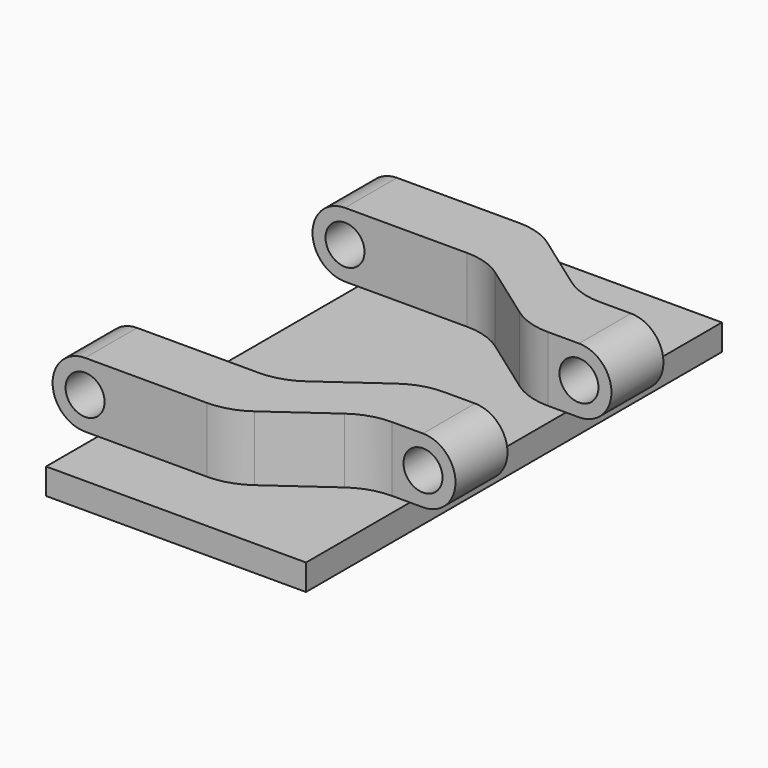
from build123d import *

# Parameters (mm, degrees)
F0_W          = 20
F0_H          = 1
F1_DEPTH      = 20
F1_DEPTH_BACK = 20
F3_DEPTH      = 40
F5_DEPTH      = 5
F7_R          = 1.5
F8_DEPTH      = 20.001
F8_DEPTH_BACK = 20.001
F9_R          = 5


# Not quite as in the source:
# - a pattern or mirror of a feature is missing from the dataset's text; its kind, count and spacing are read off the source's solid


with BuildPart() as f1:
    # F0 (on Front) → F1 (new body, two sides)
    with BuildSketch(Plane.XZ) as f1_sk:
        with Locations((0, -0.5)):
            Rectangle(F0_W, F0_H)
    extrude(amount=F1_DEPTH)
    extrude(f1_sk.sketch, amount=-F1_DEPTH_BACK)

    # F2 (on face) → F3 (join, through all)
    with BuildSketch(Plane(origin=(0, 20, 0), x_dir=(-1, 0, 0), z_dir=(0, 1, 0))):
        with BuildLine():
            Line((10, 1), (11, 1))
            ThreePointArc((11, 1), (13.5, 3.5), (11, 6))
            Line((11, 6), (0, 6))
            Line((0, 6), (-11, 6))
            ThreePointArc((-11, 6), (-13.5, 3.5), (-11, 1))
            Line((-11, 1), (-10, 1))
            Line((-10, 1), (-10, 0))
            Line((-10, 0), (0, 0))
            Line((0, 0), (10, 0))
            Line((10, 0), (10, 1))
        make_face()
    extrude(amount=-F3_DEPTH)

    # F4 (on face) → F5 (cut, through all)
    with BuildSketch(Plane.XY.offset(6)):
        Polygon((0, -15), (-13.5, -15), (-13.5, -20), (13.5, -20), (13.5, -10), (7, -10), align=None)
        Polygon((-13.5, 0), (-13.5, -10), (0, -10), (7, -5), (13.5, -5), (13.5, 0), align=None)
    f5 = extrude(amount=-F5_DEPTH, mode=Mode.SUBTRACT)

    # F5_copies: F5 across plane
    add(f5.mirror(Plane.ZX), mode=Mode.SUBTRACT)

    # F7 (on offset) → F8 (cut, two sides)
    with BuildSketch(Plane.XZ) as f8_sk:
        with Locations((11, 3.5)):
            Circle(F7_R)
        with Locations((-11, 3.5)):
            Circle(F7_R)
    extrude(amount=-F8_DEPTH, mode=Mode.SUBTRACT)
    extrude(f8_sk.sketch, amount=F8_DEPTH_BACK, mode=Mode.SUBTRACT)

    # F9
    f9_edges = [f1.edges().sort_by_distance(p)[0] for p in [
        (0, -15, 3.5),
        (0, -10, 3.5),
        (7, -5, 3.5),
        (7, -10, 3.5),
        (7, 10, 3.5),
        (0, 15, 3.5),
        (0, 10, 3.5),
        (7, 5, 3.5),
    ]]
    fillet(f9_edges, radius=F9_R)


solid = f1.part
